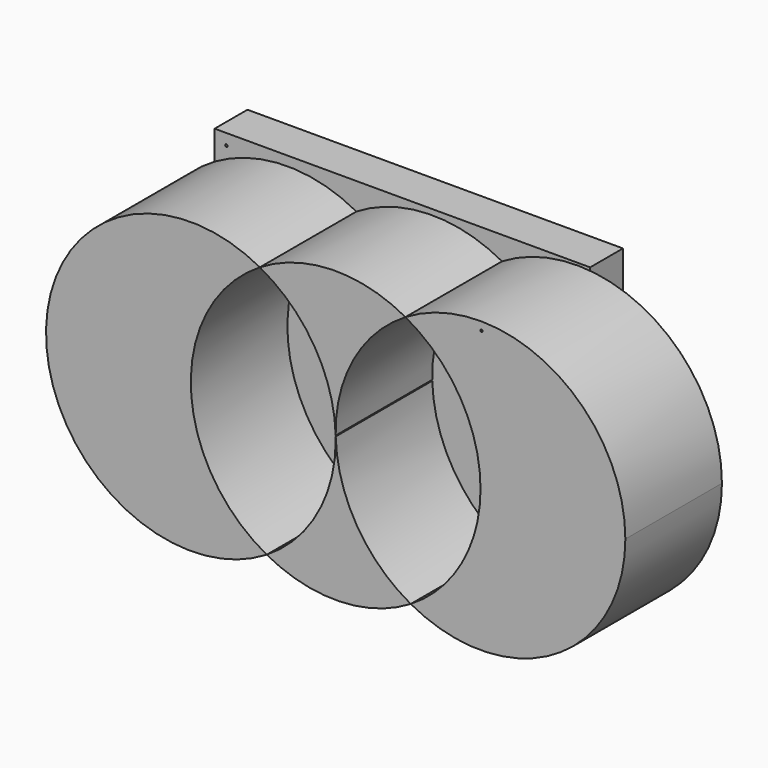
from build123d import *

# Parameters (mm, degrees)
F1_DEPTH = 25
F2_W     = 77.7685903013
F2_H     = 61.3984446973
F3_DEPTH = 8.5
F4_R     = 0.25
F5_DEPTH = 52.9


with BuildPart() as f1:
    # F0 (on Front) → F1 (new body)
    with BuildSketch(Plane.XZ):
        with BuildLine():
            ThreePointArc((-24.6252371606, 64.7749764202), (-68.899377051, 37.5757018533), (-23.2070443664, 12.832809261))
            ThreePointArc((-23.2070443664, 12.832809261), (-38.9105528593, 38.3944958448), (-24.6252371606, 64.7749764202))
        make_face()
    extrude(amount=F1_DEPTH)


with BuildPart() as f1b:
    # F0 (on Front) → F1, piece 2 (new body)
    with BuildSketch(Plane.XZ):
        with BuildLine():
            ThreePointArc((21.0782713324, 39.2132898363), (17.2153351945, 24.4873300147), (6.6213451544, 13.553733017))
            ThreePointArc((6.6213451544, 13.553733017), (36.3440176728, 14.0226209778), (51.0716362988, 39.8442082095))
            ThreePointArc((51.0716362988, 39.8442082095), (35.7975961204, 65.9812720716), (5.5285624767, 65.5037650288))
            ThreePointArc((5.5285624767, 65.5037650288), (16.8998585641, 54.4856712104), (21.0782713324, 39.2132898363))
        make_face()
    extrude(amount=F1_DEPTH)


with BuildPart() as f1c:
    # F0 (on Front) → F1, piece 3 (new body)
    with BuildSketch(Plane.XZ):
        with BuildLine():
            ThreePointArc((-24.6252371606, 64.7749764202), (-13.3488662754, 54.0980043378), (-8.9217286676, 39.2132898363))
            ThreePointArc((-8.9217286676, 39.2132898363), (-5.2188388937, 54.2944993538), (5.5285624767, 65.5037650288))
            ThreePointArc((5.5285624767, 65.5037650288), (-9.6465884056, 69.2045315305), (-24.6252371606, 64.7749764202))
        make_face()
    extrude(amount=F1_DEPTH)


with BuildPart() as f1d:
    # F0 (on Front) → F1, piece 4 (new body)
    with BuildSketch(Plane.XZ):
        with BuildLine():
            ThreePointArc((-8.9171878929, 39.025414218), (-8.9122116636, 38.7099724752), (-8.9105528593, 38.3944958448))
            ThreePointArc((-8.9105528593, 38.3944958448), (-12.7274929275, 23.7504741088), (-23.2070443664, 12.832809261))
            ThreePointArc((-23.2070443664, 12.832809261), (-8.1968689297, 9.2220481421), (6.6213451544, 13.553733017))
            ThreePointArc((6.6213451544, 13.553733017), (-4.5391110305, 24.2208404151), (-8.9171878929, 39.025414218))
        make_face()
    extrude(amount=F1_DEPTH)


with BuildPart() as f3:
    # F2 (on Front) → F3 (new body)
    with BuildSketch(Plane.XZ):
        with Locations((-15.1060316712, 39.6397346631)):
            Rectangle(F2_W, F2_H)
    extrude(amount=-F3_DEPTH)


with BuildPart() as f5_tool:
    # F4 (on face) → F5 (new body)
    with BuildSketch(Plane(origin=(0, 8.5, 0), x_dir=(-1, 0, 0), z_dir=(0, 1, 0))):
        with Locations((-21.2886072695, 68.143799901)):
            Circle(F4_R)
        with Locations((51.5504516661, 68.0448934436)):
            Circle(F4_R)
    extrude(amount=-F5_DEPTH)


with BuildPart() as f1b_1:
    add(f1b.part)

    # F5: cut by f5_tool
    add(f5_tool.part, mode=Mode.SUBTRACT)


with BuildPart() as f3_1:
    add(f3.part)

    # F5: cut by f5_tool
    add(f5_tool.part, mode=Mode.SUBTRACT)


solid = Compound([f1.part, f1c.part, f1d.part, f1b_1.part, f3_1.part])
